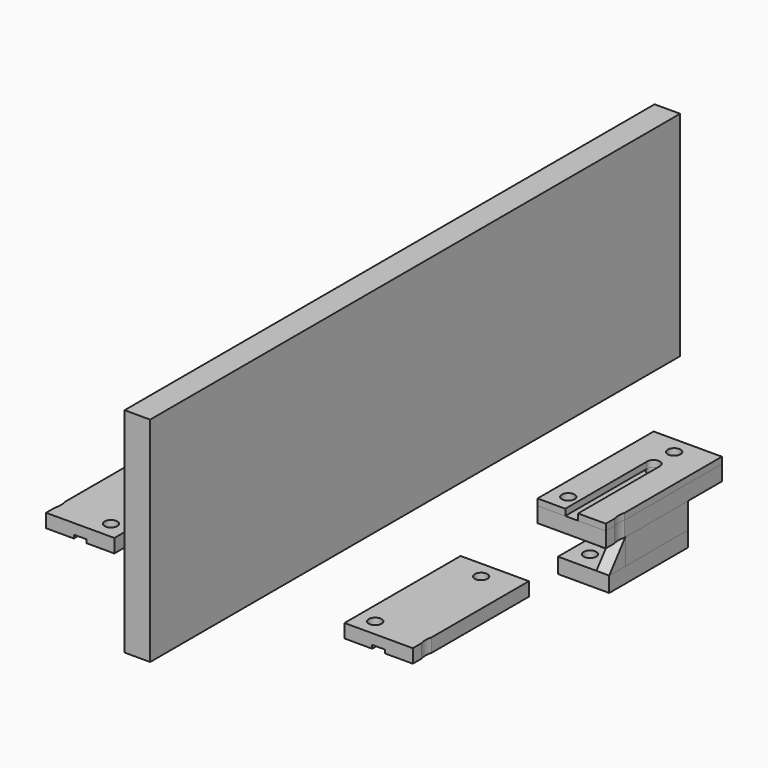
from build123d import *
from build123d import SkipClean  # not in build123d's __all__

# Parameters (mm, degrees)
F0_R      = 0.75
F1_DEPTH  = 1.8
F2_R      = 0.75
F3_DEPTH  = 0.75
F5_DEPTH  = 1.2
F6_DEPTH  = 0.4
F4_W      = 1.8
F4_H      = 9.15
F7_DEPTH  = 3
F8_R      = 0.75
F8_W      = 1.8
F8_H      = 9.15
F9_DEPTH  = 1.8
F11_DEPTH = 1.5
F0_W      = 2.992650494
F0_H      = 77.5951314718
F12_DEPTH = 25


# Not quite as in the source:
# - a feature names something its author has since deleted; it is built from what else it names


with BuildPart() as f1:
    # F0 (on Top) → F1 (new body)
    with BuildSketch(Plane.XY):
        with BuildLine():
            Line((2.790238331, 8.9906946085), (-5.209761669, 8.9906946085))
            Line((-5.209761669, 8.9906946085), (-5.209761669, -5.2593053915))
            ThreePointArc((-5.209761669, -5.2593053915), (-5.1019243438, -6.0093053915), (-5.209761669, -6.7593053915))
            Line((-5.209761669, -6.7593053915), (-5.209761669, -8.0093053915))
            Line((-5.209761669, -8.0093053915), (2.790238331, -8.0093053915))
            Line((2.790238331, -8.0093053915), (2.790238331, 8.9906946085))
        make_face()
        with Locations((0.790238331, -6.0093053915)):
            Circle(F0_R, mode=Mode.SUBTRACT)
        with Locations((-1.209761669, 3.9906946085)):
            Circle(F0_R, mode=Mode.SUBTRACT)
        with Locations((-1.209761669, 6.9906946085)):
            Circle(F0_R, mode=Mode.SUBTRACT)
    extrude(amount=F1_DEPTH)

    # F2 (on face) → F3 (join)
    with BuildSketch(Plane.XY.offset(1.8)):
        with BuildLine():
            ThreePointArc((-1.959761669, 3.9906946085), (-1.209761669, 4.7406946085), (-0.459761669, 3.9906946085))
            Line((-0.459761669, 3.9906946085), (-0.459761669, -8.0093053915))
            Line((-0.459761669, -8.0093053915), (2.790238331, -8.0093053915))
            Line((2.790238331, -8.0093053915), (2.790238331, 8.9906946085))
            Line((2.790238331, 8.9906946085), (-5.209761669, 8.9906946085))
            Line((-5.209761669, 8.9906946085), (-5.209761669, -5.2593053915))
            ThreePointArc((-5.209761669, -5.2593053915), (-5.1019243438, -6.0093053915), (-5.209761669, -6.7593053915))
            Line((-5.209761669, -6.7593053915), (-5.209761669, -8.0093053915))
            Line((-5.209761669, -8.0093053915), (-1.959761669, -8.0093053915))
            Line((-1.959761669, -8.0093053915), (-1.959761669, 3.9906946085))
        make_face()
        with Locations((0.790238331, -6.0093053915)):
            Circle(F2_R, mode=Mode.SUBTRACT)
        with Locations((-1.209761669, 6.9906946085)):
            Circle(F2_R, mode=Mode.SUBTRACT)
    with SkipClean():  # cleaning this boolean's faces spoils the solid; the shape is the same uncleaned
        extrude(amount=F3_DEPTH)

    # F4 (on face) → F7 (join)
    with BuildSketch(Plane(origin=(0, 0, 0), x_dir=(1, 0, 0), z_dir=(0, 0, -1))):
        with Locations((-4.309761669, 0.5843053915)):
            Rectangle(F4_W, F4_H)
    with SkipClean():  # cleaning this boolean's faces spoils the solid; the shape is the same uncleaned
        extrude(amount=F7_DEPTH)

    # F8 (on face) → F9 (join)
    with BuildSketch(Plane(origin=(0, 0, -3), x_dir=(1, 0, 0), z_dir=(0, 0, -1))):
        Polygon((-3.409761669, 5.1593053915), (-3.409761669, -3.9906946085), (0.790238331, -3.9906946085), (0.790238331, 7.5093053915), (-5.209761669, 7.5093053915), (-5.209761669, 5.1593053915), align=None)
        with Locations((-1.196700694, -2.1906946085)):
            Circle(F8_R, mode=Mode.SUBTRACT)
        with Locations((-1.196700694, 0.3093053915)):
            Circle(F8_R, mode=Mode.SUBTRACT)
        with Locations((-1.196700694, 2.8093053915)):
            Circle(F8_R, mode=Mode.SUBTRACT)
        with Locations((-1.196700694, 5.3093053915)):
            Circle(F8_R, mode=Mode.SUBTRACT)
        with Locations((-4.309761669, 0.5843053915)):
            Rectangle(F8_W, F8_H)
    with SkipClean():  # cleaning this boolean's faces spoils the solid; the shape is the same uncleaned
        extrude(amount=F9_DEPTH)

    # F10 (on face) → F11 (join)
    with BuildSketch(Plane(origin=(-5.209761669, 0, 0), x_dir=(0, -1, 0), z_dir=(-1, 0, 0))):
        Polygon((5.1593053915, 0), (5.1593053915, -3), (7.5093053915, -3), align=None)
    with SkipClean():  # cleaning this boolean's faces spoils the solid; the shape is the same uncleaned
        extrude(amount=-F11_DEPTH)


with BuildPart() as f5:
    # F0 (on Top) → F5 (new body)
    with BuildSketch(Plane.XY):
        with BuildLine():
            Line((-5.209761669, -35.0220153915), (-5.209761669, -36.2720153915))
            Line((-5.209761669, -36.2720153915), (-1.959761669, -36.2720153915))
            Line((-1.959761669, -36.2720153915), (-1.959761669, -24.2720153915))
            ThreePointArc((-1.959761669, -24.2720153915), (-1.209761669, -23.5220153915), (-0.459761669, -24.2720153915))
            Line((-0.459761669, -24.2720153915), (-0.459761669, -36.2720153915))
            Line((-0.459761669, -36.2720153915), (2.790238331, -36.2720153915))
            Line((2.790238331, -36.2720153915), (2.790238331, -19.2720153915))
            Line((2.790238331, -19.2720153915), (-5.209761669, -19.2720153915))
            Line((-5.209761669, -19.2720153915), (-5.209761669, -33.5220153915))
            ThreePointArc((-5.209761669, -33.5220153915), (-5.1019243438, -34.2720153915), (-5.209761669, -35.0220153915))
        make_face()
        with Locations((0.790238331, -34.2720153915)):
            Circle(F0_R, mode=Mode.SUBTRACT)
        with Locations((-1.209761669, -21.2720153915)):
            Circle(F0_R, mode=Mode.SUBTRACT)
        with BuildLine():
            Line((-1.959761669, -24.2720153915), (-1.959761669, -36.2720153915))
            Line((-1.959761669, -36.2720153915), (-0.459761669, -36.2720153915))
            Line((-0.459761669, -36.2720153915), (-0.459761669, -24.2720153915))
            ThreePointArc((-0.459761669, -24.2720153915), (-1.209761669, -25.0220153915), (-1.959761669, -24.2720153915))
        make_face()
        with BuildLine():
            ThreePointArc((-0.459761669, -24.2720153915), (-1.209761669, -23.5220153915), (-1.959761669, -24.2720153915))
            ThreePointArc((-1.959761669, -24.2720153915), (-1.209761669, -25.0220153915), (-0.459761669, -24.2720153915))
        make_face()
    extrude(amount=F5_DEPTH)

    # F0 (on Top) → F6 (join)
    with BuildSketch(Plane.XY):
        with BuildLine():
            Line((-5.209761669, -35.0220153915), (-5.209761669, -36.2720153915))
            Line((-5.209761669, -36.2720153915), (-1.959761669, -36.2720153915))
            Line((-1.959761669, -36.2720153915), (-1.959761669, -24.2720153915))
            ThreePointArc((-1.959761669, -24.2720153915), (-1.209761669, -23.5220153915), (-0.459761669, -24.2720153915))
            Line((-0.459761669, -24.2720153915), (-0.459761669, -36.2720153915))
            Line((-0.459761669, -36.2720153915), (2.790238331, -36.2720153915))
            Line((2.790238331, -36.2720153915), (2.790238331, -19.2720153915))
            Line((2.790238331, -19.2720153915), (-5.209761669, -19.2720153915))
            Line((-5.209761669, -19.2720153915), (-5.209761669, -33.5220153915))
            ThreePointArc((-5.209761669, -33.5220153915), (-5.1019243438, -34.2720153915), (-5.209761669, -35.0220153915))
        make_face()
        with Locations((0.790238331, -34.2720153915)):
            Circle(F0_R, mode=Mode.SUBTRACT)
        with Locations((-1.209761669, -21.2720153915)):
            Circle(F0_R, mode=Mode.SUBTRACT)
    extrude(amount=-F6_DEPTH)


with BuildPart() as f12:
    # F0 (on Top) → F12 (new body)
    with BuildSketch(Plane.XY):
        with Locations((17.7631499246, -12.824180536)):
            Rectangle(F0_W, F0_H)
    extrude(amount=F12_DEPTH)


with BuildPart() as f13_1:
    # F13: instance of F5
    add(f5.part.mirror(Plane(origin=(16.2668246776, -12.824180536, 12.5), x_dir=(0, -1, 0), z_dir=(-1, 0, 0))), clean=False)


with BuildPart() as f13_2:
    # F13: instance of F1
    add(f1.part.mirror(Plane(origin=(16.2668246776, -12.824180536, 12.5), x_dir=(0, -1, 0), z_dir=(-1, 0, 0))), clean=False)


solid = Compound([f1.part, f5.part, f12.part, f13_1.part, f13_2.part])
